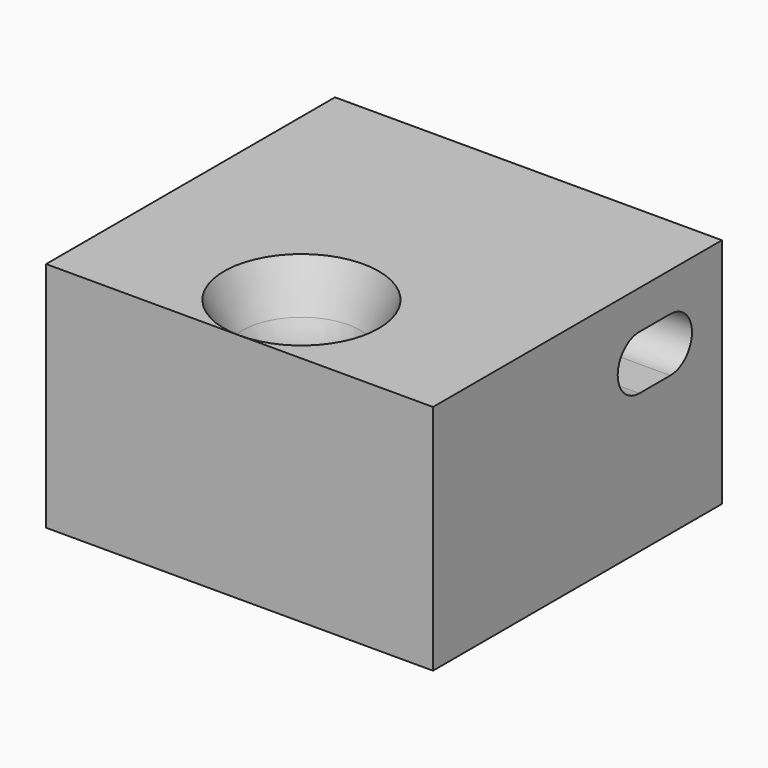
from build123d import *

# Parameters (mm, degrees)
F0_W     = 30
F0_H     = 28
F0_R     = 4
F1_DEPTH = 18
F4_DEPTH = 40
F6_R     = 8
F7_R     = 8


# Not quite as in the source:
# - a fillet or chamfer that OpenCascade refuses, or shapes differently, is made with other operations: its cross-section is extruded or revolved along the edge and cut away or added


with BuildPart() as f1:
    # F0 (on Top) → F1 (new body)
    with BuildSketch(Plane.XY):
        with Locations((-30.3913680837, 12.4760417278)):
            Rectangle(F0_W, F0_H)
        with Locations((-30.3913680837, 4.4760417278)):
            Circle(F0_R, mode=Mode.SUBTRACT)
    extrude(amount=F1_DEPTH)

    # F2: chamfer of 2 x 8 on 1 edges, made by hand

    # F2_s1 → F2_t2 (revolve, cut)
    with BuildSketch(Plane.XZ.offset(-4.4760417278)):
        Polygon((-26.3913680837, 8), (-24.3913680837, 0), (-26.3913680837, 0), align=None)
    revolve(axis=Axis((-30.3913680837, 4.4760417278, 0), (0, 0, 1)), mode=Mode.SUBTRACT)

    # F3 (on face) → F4 (cut)
    with BuildSketch(Plane.YZ.offset(-15.3913680837)):
        with BuildLine():
            Line((18.4760417278, 10.8), (21.4760417278, 10.8))
            ThreePointArc((21.4760417278, 10.8), (23.5760417278, 12.9), (21.4760417278, 15))
            Line((21.4760417278, 15), (18.4760417278, 15))
            ThreePointArc((18.4760417278, 15), (16.3760417278, 12.9), (18.4760417278, 10.8))
        make_face()
    extrude(amount=-F4_DEPTH, mode=Mode.SUBTRACT)

    # F5: chamfer of 5 x 2 on 1 edges, made by hand

    # F5_s1 → F5_t2 (revolve, cut)
    with BuildSketch(Plane.XZ.offset(-4.4760417278)):
        Polygon((-24.3913680837, 18), (-26.3913680837, 13), (-26.3913680837, 18), align=None)
    revolve(axis=Axis((-30.3913680837, 4.4760417278, 18), (0, 0, 1)), mode=Mode.SUBTRACT)

    # F6
    f6_edges = [f1.edges().sort_by_distance(p)[0] for p in [
        (-34.391368, 4.476042, 13),
    ]]
    fillet(f6_edges, radius=F6_R)

    # F7
    f7_edges = [f1.edges().sort_by_distance(p)[0] for p in [
        (-34.391368, 4.476042, 8),
    ]]
    fillet(f7_edges, radius=F7_R)


solid = f1.part
